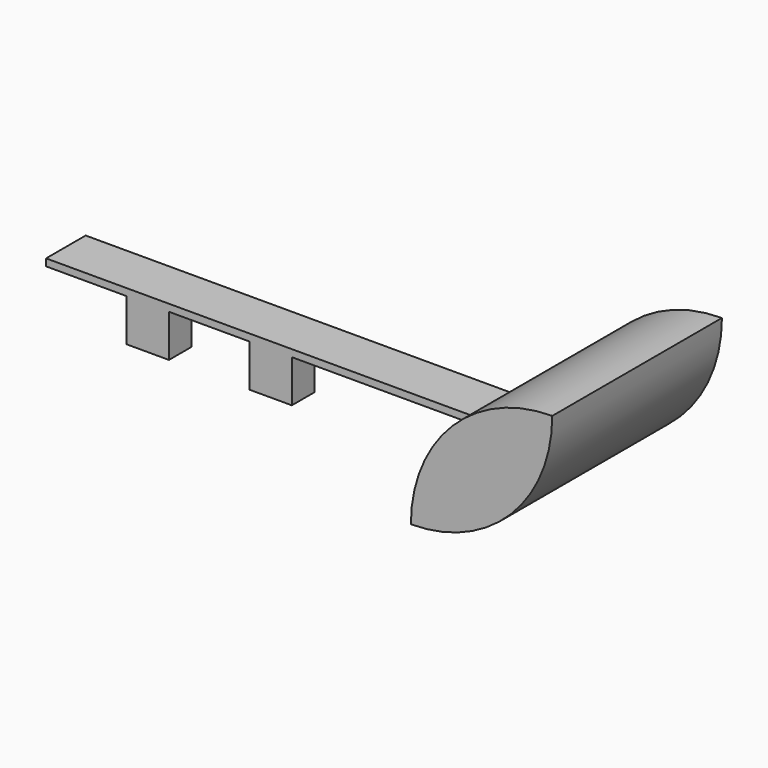
from build123d import *

# Parameters (mm, degrees)
F1_DEPTH = 1.27
F0_W     = 7.62
F0_H     = 5.08
F2_DEPTH = 7.62
F3_DEPTH = 1.27
F4_DEPTH = 25.4
F5_R     = 25.39999
F6_R     = 25.39999


# Not quite as in the source:
# - a fillet or chamfer is up to 0.001 mm smaller than in the source, because OpenCascade refuses the exact size


with BuildPart() as f1:
    # F0 (on Top) → F1 (new body)
    with BuildSketch(Plane.XY):
        Polygon((-56.5321096511, 32.319452062), (-145.4321096511, 32.319452062), (-145.4321096511, 23.429452062), (-130.9795096511, 23.429452062), (-130.9795096511, 28.509452062), (-123.3595096511, 28.509452062), (-123.3595096511, 23.429452062), (-108.9069096511, 23.429452062), (-108.9069096511, 28.509452062), (-101.2869096511, 28.509452062), (-101.2869096511, 23.429452062), (-56.5321096511, 23.429452062), align=None)
    extrude(amount=F1_DEPTH)



with BuildPart() as f2:
    # F0 (on Top) → F2 (new body)
    with BuildSketch(Plane.XY):
        with Locations((-127.1695096511, 25.969452062)):
            Rectangle(F0_W, F0_H)
    extrude(amount=-F2_DEPTH)


with BuildPart() as f2b:
    # F0 (on Top) → F2, piece 2 (new body)
    with BuildSketch(Plane.XY):
        with Locations((-105.0969096511, 25.969452062)):
            Rectangle(F0_W, F0_H)
    extrude(amount=-F2_DEPTH)


with BuildPart() as f1_1:
    add(f1.part)

    add(f2.part)  # F3 merges F2

    add(f2b.part)  # F3 merges F2b
    # F0 (on Top) → F3 (join)
    with BuildSketch(Plane.XY):
        with Locations((-127.1695096511, 25.969452062)):
            Rectangle(F0_W, F0_H)
        with Locations((-105.0969096511, 25.969452062)):
            Rectangle(F0_W, F0_H)
    extrude(amount=F3_DEPTH)

    # F0 (on Top) → F4 (join)
    with BuildSketch(Plane.XY):
        Polygon((-31.1321096511, 32.319452062), (-56.5321096511, 32.319452062), (-56.5321096511, 23.429452062), (-56.5321096511, -5.780547938), (-31.1321096511, -5.780547938), align=None)
    extrude(amount=F4_DEPTH)

    # F5 (radius 25.4 in the source; OpenCascade refuses exactly that, so slightly less here)
    f5_edges = [f1_1.edges().sort_by_distance(p)[0] for p in [
        (-31.13211, 13.269452, 0),
    ]]
    fillet(f5_edges, radius=F5_R)

    # F6 (radius 25.4 in the source; OpenCascade refuses exactly that, so slightly less here)
    f6_edges = [f1_1.edges().sort_by_distance(p)[0] for p in [
        (-56.53211, 13.269452, 25.4),
    ]]
    fillet(f6_edges, radius=F6_R)


solid = f1_1.part
